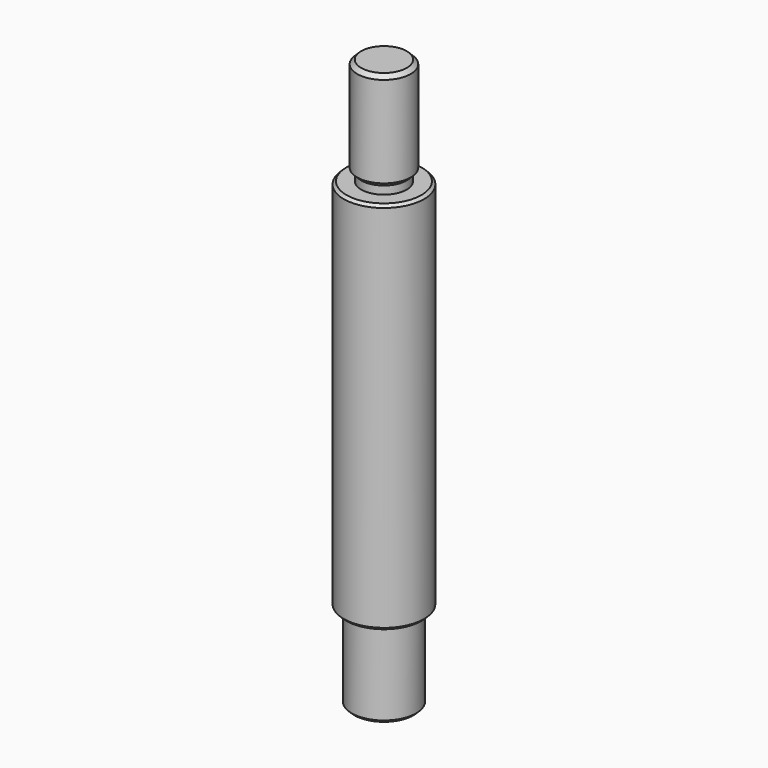
from build123d import *

# Parameters (mm, degrees)
F2_SIZE = 0.74999
F3_SIZE = 0.5


# Not quite as in the source:
# - a fillet or chamfer is up to 0.001 mm smaller than in the source, because OpenCascade refuses the exact size


with BuildPart() as f1:
    # F0 (on Front) → F1 (revolve)
    with BuildSketch(Plane.XZ):
        Polygon((-6, 0), (0, 0), (0, 106), (-5, 106), (-5, 87.5), (-4.25, 87.5), (-4.25, 86), (-5, 86), (-7.5, 86), (-7.5, 16), (-6, 16), (-6, 14.25), align=None)
    revolve(axis=Axis((0, 0, 53), (0, 0, -1)))

    # F2 (size 0.75 in the source; OpenCascade refuses exactly that, so slightly less here)
    f2_edges = [f1.edges().sort_by_distance(p)[0] for p in [
        (5, 0, 106),
        (5, 0, 87.5),
        (-5, 0, 96.75),
    ]]
    chamfer(f2_edges, length=F2_SIZE)

    # F3
    f3_edges = [f1.edges().sort_by_distance(p)[0] for p in [
        (7.5, 0, 86),
        (7.5, 0, 16),
        (-7.5, 0, 51),
        (6, 0, 0),
        (6, 0, 16),
    ]]
    chamfer(f3_edges, length=F3_SIZE)


solid = f1.part
